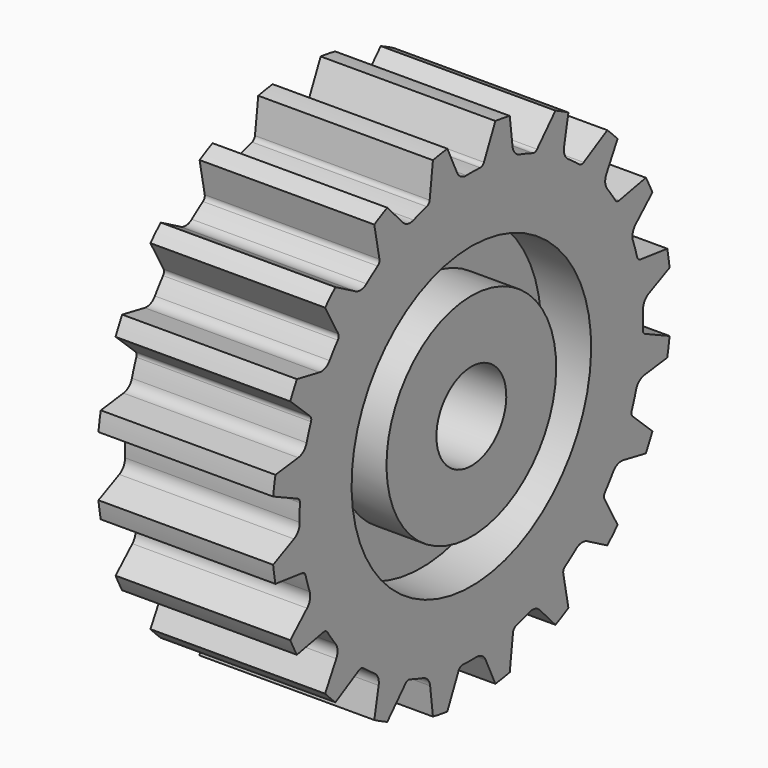
from build123d import *

# Parameters (mm, degrees)
F3_DEPTH        = 70.001
F3_COPIES_COUNT = 20


# Not quite as in the source:
# - a feature of the source that left no trace in its solid (it failed there, or was rolled back) is left out
# - a pattern or mirror of a feature is missing from the dataset's text; its kind, count and spacing are read off the source's solid


with BuildPart() as f1:
    # F0 (on Front) → F1 (revolve)
    with BuildSketch(Plane.XZ):
        Polygon((35, -20), (35, 20), (-35, 20), (-35, -20), (-15, -20), (-15, -37.5), (-35, -37.5), (-35, -62.5), (35, -62.5), (35, -37.5), (15, -37.5), (15, -20), align=None)
    revolve(axis=Axis((-7.5, 0, -80), (-1, 0, 0)))

    # F2 (on face) → F3 (cut, through all)
    with BuildSketch(Plane.YZ.offset(35)):
        with BuildLine():
            ThreePointArc((-2.4875303205, 5.9552673354), (0.9594167449, 5.9859018055), (4.4048221019, 5.878363585))
            ThreePointArc((4.4048221019, 5.878363585), (5.5383005859, 6.1619770528), (6.3198858178, 7.0305014326))
            Line((6.3198858178, 7.0305014326), (12.0290632191, 19.2738718801))
            ThreePointArc((12.0290632191, 19.2738718801), (0, 20), (-12.0290632191, 19.2738718801))
            Line((-12.0290632191, 19.2738718801), (-7.1637078206, 8.8400835574))
            ThreePointArc((-7.1637078206, 8.8400835574), (-5.2573859952, 6.6977976646), (-2.4875303205, 5.9552673354))
        make_face()
    f3 = extrude(amount=-F3_DEPTH, mode=Mode.SUBTRACT)

    # F3_copies: F3 ×20 about axis
    f3_copies_axis = Axis((0, 0, -80), (1, 0, 0))
    for i in range(1, F3_COPIES_COUNT):
        add(f3.rotate(f3_copies_axis, i * 360 / F3_COPIES_COUNT), mode=Mode.SUBTRACT)


solid = f1.part
